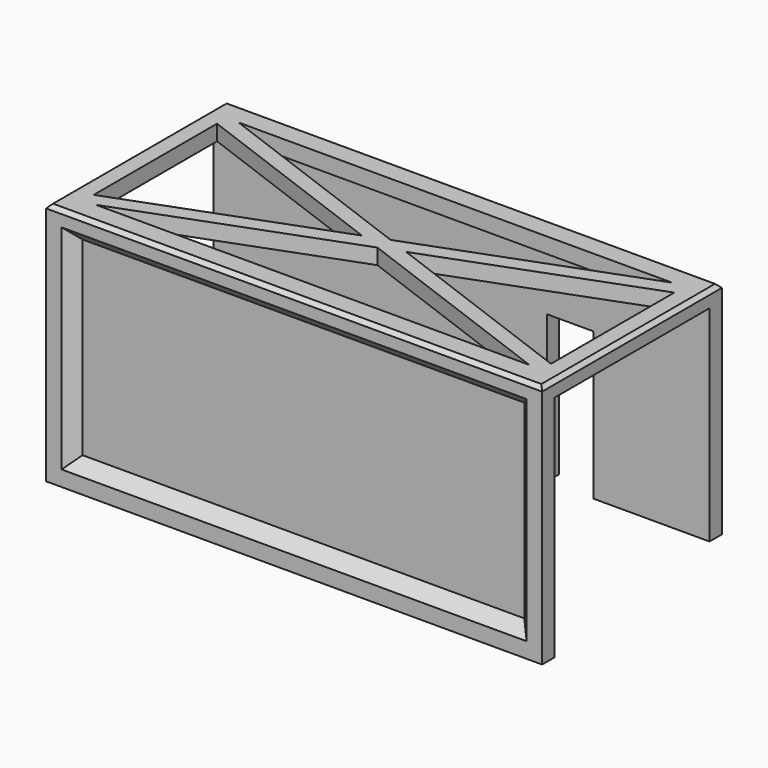
from build123d import *

# Parameters (mm, degrees)
F1_DEPTH  = 32
F3_DEPTH  = 1.5
F2_W      = 6
F2_H      = 19
F4_DEPTH  = 2
F5_W      = 60
F5_H      = 27.5
F6_DEPTH  = 1.5
F7_SIZE   = 1.49999
F8_SIZE   = 0.5
F10_DEPTH = 2


# Not quite as in the source:
# - a fillet or chamfer is up to 0.001 mm smaller than in the source, because OpenCascade refuses the exact size


with BuildPart() as f1:
    # F0 (on Right) → F1 (new body, symmetric)
    with BuildSketch(Plane.YZ):
        Polygon((-12.5, 0), (-12.5, 29.5), (12.5, 29.5), (12.5, 3), (14.5, 3), (14.5, 31.5), (-14.5, 31.5), (-14.5, 0), align=None)
    extrude(amount=F1_DEPTH, both=True)

    # F2 (on face) → F3 (cut)
    with BuildSketch(Plane(origin=(0, 14.5, 0), x_dir=(-1, 0, 0), z_dir=(0, 1, 0))):
        Polygon((-9, 5), (30, 5), (30, 29.5), (-30, 29.5), (-30, 5), (-19, 5), (-19, 24), (-9, 24), align=None)
    extrude(amount=-F3_DEPTH, mode=Mode.SUBTRACT)

    # F2 (on face) → F4 (cut)
    with BuildSketch(Plane(origin=(0, 14.5, 0), x_dir=(-1, 0, 0), z_dir=(0, 1, 0))):
        with Locations((-14, 12.5)):
            Rectangle(F2_W, F2_H)
    extrude(amount=-F4_DEPTH, mode=Mode.SUBTRACT)

    # F5 (on face) → F6 (cut)
    with BuildSketch(Plane.XZ.offset(14.5)):
        with Locations((0, 15.75)):
            Rectangle(F5_W, F5_H)
    extrude(amount=-F6_DEPTH, mode=Mode.SUBTRACT)

    # F7 (size 1.5 in the source; OpenCascade refuses exactly that, so slightly less here)
    f7_edges = [f1.edges().sort_by_distance(p)[0] for p in [
        (-30, 13, 17.25),
        (0, 13, 29.5),
        (30, 13, 17.25),
        (9, 13, 14.5),
        (-10.5, 13, 5),
        (24.5, 13, 5),
        (19, 13, 14.5),
        (14, 13, 24),
        (0, -13, 29.5),
        (-30, -13, 15.75),
        (0, -13, 2),
        (30, -13, 15.75),
    ]]
    chamfer(f7_edges, length=F7_SIZE)

    # F8
    f8_edges = [f1.edges().sort_by_distance(p)[0] for p in [
        (0, 14.5, 31.5),
        (0, -14.5, 31.5),
        (32, 0, 31.5),
        (-32, 0, 31.5),
    ]]
    chamfer(f8_edges, length=F8_SIZE)

    # F9 (on face) → F10 (cut)
    with BuildSketch(Plane.XY.offset(31.5)):
        Polygon((27.9455012138, 11.5), (-27.9455012138, 11.5), (0, 1.0674114154), align=None)
        Polygon((-2.8592469416, 0), (-29.5, 9.9455012138), (-29.5, -9.9455012138), align=None)
        Polygon((0, -1.0674114154), (-27.9455012138, -11.5), (27.9455012138, -11.5), align=None)
        Polygon((29.5, -9.9455012138), (29.5, 9.9455012138), (2.8592469416, 0), align=None)
    extrude(amount=-F10_DEPTH, mode=Mode.SUBTRACT)


solid = f1.part
